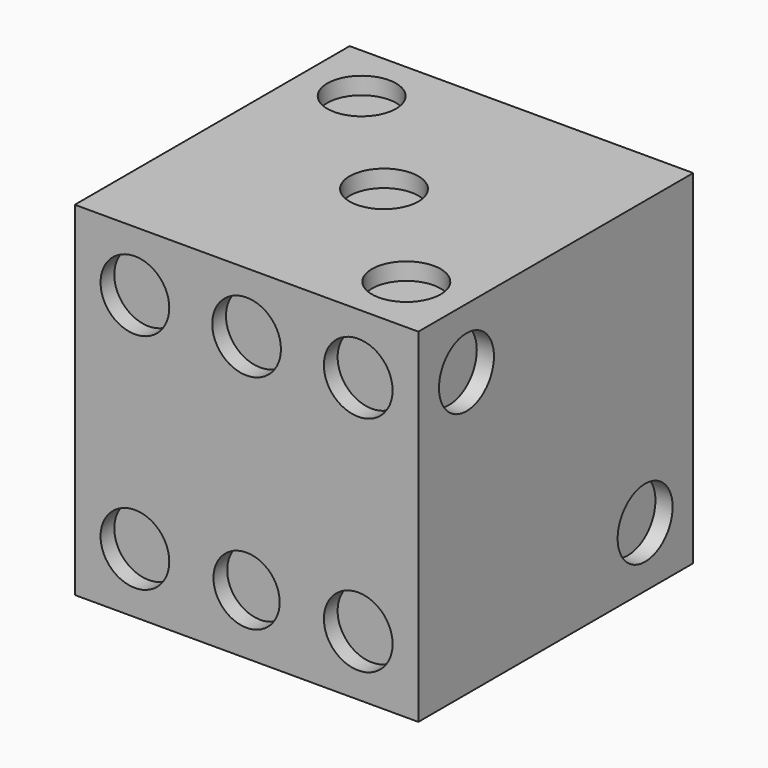
from build123d import *

# Parameters (mm, degrees)
F0_W      = 127
F0_H      = 127
F1_DEPTH  = 127
F2_R      = 12.7
F3_DEPTH  = 6.35
F4_R      = 12.7
F5_DEPTH  = 6.35
F6_R      = 12.7
F7_DEPTH  = 6.35
F8_R      = 12.7
F9_DEPTH  = 6.35
F10_R     = 12.7
F11_DEPTH = 6.35
F12_R     = 12.7
F13_DEPTH = 6.35
F14_R     = 12.7
F15_DEPTH = 6.35
F16_R     = 12.7
F17_DEPTH = 6.35
F18_R     = 12.7
F19_DEPTH = 6.35
F20_R     = 12.2418661496
F21_DEPTH = 6.35
F22_R     = 12.7
F23_DEPTH = 6.35
F25_R     = 12.7
F26_DEPTH = 6.35
F27_R     = 12.7
F28_DEPTH = 6.35
F29_R     = 12.7
F30_DEPTH = 6.35
F31_R     = 12.7
F32_DEPTH = 6.35
F33_R     = 12.7
F34_DEPTH = 6.35
F35_R     = 12.7
F36_DEPTH = 6.35
F37_R     = 12.7
F38_DEPTH = 6.35
F39_R     = 12.7
F40_DEPTH = 6.35
F41_R     = 12.7
F42_DEPTH = 6.35
F43_R     = 12.7
F44_DEPTH = 6.35


# Not quite as in the source:
# - a length typed as a fraction of an inch, garbled in the dataset ("3 / 203.2 mm" for 3/8 in), is restored


with BuildPart() as f1:
    # F0 (on Right) → F1 (new body)
    with BuildSketch(Plane.YZ):
        with Locations((-2.1555427632, -5.2600353956)):
            Rectangle(F0_W, F0_H)
    extrude(amount=F1_DEPTH)

    # F2 (on face) → F3 (cut)
    with BuildSketch(Plane(origin=(0, 61.3444572368, 0), x_dir=(-1, 0, 0), z_dir=(0, 1, 0))):
        with Locations((-63.2817981055, -5.2596604964)):
            Circle(F2_R)
    extrude(amount=-F3_DEPTH, mode=Mode.SUBTRACT)

    # F4 (on face) → F5 (cut)
    with BuildSketch(Plane(origin=(0, 0, 0), x_dir=(0, -1, 0), z_dir=(-1, 0, 0))):
        with Locations((2.032, -6.35)):
            Circle(F4_R)
    extrude(amount=-F5_DEPTH, mode=Mode.SUBTRACT)

    # F6 (on face) → F7 (cut)
    with BuildSketch(Plane(origin=(0, 0, 0), x_dir=(0, -1, 0), z_dir=(-1, 0, 0))):
        with Locations((-39.1194572368, 36.0149646044)):
            Circle(F6_R)
    extrude(amount=-F7_DEPTH, mode=Mode.SUBTRACT)

    # F8 (on face) → F9 (cut)
    with BuildSketch(Plane(origin=(0, 0, 0), x_dir=(0, -1, 0), z_dir=(-1, 0, 0))):
        with Locations((43.4305427632, 36.0149646044)):
            Circle(F8_R)
    extrude(amount=-F9_DEPTH, mode=Mode.SUBTRACT)

    # F10 (on face) → F11 (cut)
    with BuildSketch(Plane(origin=(0, 0, 0), x_dir=(0, -1, 0), z_dir=(-1, 0, 0))):
        with Locations((-39.1194572368, -46.5350353956)):
            Circle(F10_R)
    extrude(amount=-F11_DEPTH, mode=Mode.SUBTRACT)

    # F12 (on face) → F13 (cut)
    with BuildSketch(Plane(origin=(0, 0, 0), x_dir=(0, -1, 0), z_dir=(-1, 0, 0))):
        with Locations((43.4305427632, -46.5350353956)):
            Circle(F12_R)
    extrude(amount=-F13_DEPTH, mode=Mode.SUBTRACT)

    # F14 (on face) → F15 (cut)
    with BuildSketch(Plane.YZ.offset(127)):
        with Locations((39.1194572368, -46.5350353956)):
            Circle(F14_R)
    extrude(amount=-F15_DEPTH, mode=Mode.SUBTRACT)

    # F16 (on face) → F17 (cut)
    with BuildSketch(Plane.YZ.offset(127)):
        with Locations((-43.4305427632, 36.0149646044)):
            Circle(F16_R)
    extrude(amount=-F17_DEPTH, mode=Mode.SUBTRACT)

    # F18 (on face) → F19 (cut)
    with BuildSketch(Plane.XZ.offset(65.6555427632)):
        with Locations((104.775, -46.5350353956)):
            Circle(F18_R)
    extrude(amount=-F19_DEPTH, mode=Mode.SUBTRACT)

    # F20 (on face) → F21 (cut)
    with BuildSketch(Plane.XZ.offset(65.6555427632)):
        with Locations((63.5, -46.5350353956)):
            Circle(F20_R)
    extrude(amount=-F21_DEPTH, mode=Mode.SUBTRACT)

    # F22 (on face) → F23 (cut)
    with BuildSketch(Plane.XZ.offset(65.6555427632)):
        with Locations((22.225, -46.5350353956)):
            Circle(F22_R)
    extrude(amount=-F23_DEPTH, mode=Mode.SUBTRACT)

    # F25 (on face) → F26 (cut)
    with BuildSketch(Plane.XZ.offset(65.6555427632)):
        with Locations((104.775, 36.0149646044)):
            Circle(F25_R)
    extrude(amount=-F26_DEPTH, mode=Mode.SUBTRACT)

    # F27 (on face) → F28 (cut)
    with BuildSketch(Plane.XZ.offset(65.6555427632)):
        with Locations((63.5, 36.0149646044)):
            Circle(F27_R)
    extrude(amount=-F28_DEPTH, mode=Mode.SUBTRACT)

    # F29 (on face) → F30 (cut)
    with BuildSketch(Plane.XZ.offset(65.6555427632)):
        with Locations((22.225, 36.0149646044)):
            Circle(F29_R)
    extrude(amount=-F30_DEPTH, mode=Mode.SUBTRACT)

    # F31 (on face) → F32 (cut)
    with BuildSketch(Plane.XY.offset(58.2399646044)):
        with Locations((104.775, -43.4305427632)):
            Circle(F31_R)
    extrude(amount=-F32_DEPTH, mode=Mode.SUBTRACT)

    # F33 (on face) → F34 (cut)
    with BuildSketch(Plane.XY.offset(58.2399646044)):
        with Locations((63.5, -2.1555427632)):
            Circle(F33_R)
    extrude(amount=-F34_DEPTH, mode=Mode.SUBTRACT)

    # F35 (on face) → F36 (cut)
    with BuildSketch(Plane.XY.offset(58.2399646044)):
        with Locations((22.225, 39.1194572368)):
            Circle(F35_R)
    extrude(amount=-F36_DEPTH, mode=Mode.SUBTRACT)

    # F37 (on face) → F38 (cut)
    with BuildSketch(Plane(origin=(0, 0, -68.7600353956), x_dir=(1, 0, 0), z_dir=(0, 0, -1))):
        with Locations((104.775, 43.4305427632)):
            Circle(F37_R)
    extrude(amount=-F38_DEPTH, mode=Mode.SUBTRACT)

    # F39 (on face) → F40 (cut)
    with BuildSketch(Plane(origin=(0, 0, -68.7600353956), x_dir=(1, 0, 0), z_dir=(0, 0, -1))):
        with Locations((22.225, 43.4305427632)):
            Circle(F39_R)
    extrude(amount=-F40_DEPTH, mode=Mode.SUBTRACT)

    # F41 (on face) → F42 (cut)
    with BuildSketch(Plane(origin=(0, 0, -68.7600353956), x_dir=(1, 0, 0), z_dir=(0, 0, -1))):
        with Locations((22.225, -39.1194572368)):
            Circle(F41_R)
    extrude(amount=-F42_DEPTH, mode=Mode.SUBTRACT)

    # F43 (on face) → F44 (cut)
    with BuildSketch(Plane(origin=(0, 0, -68.7600353956), x_dir=(1, 0, 0), z_dir=(0, 0, -1))):
        with Locations((104.775, -39.1194572368)):
            Circle(F43_R)
    extrude(amount=-F44_DEPTH, mode=Mode.SUBTRACT)


solid = f1.part
